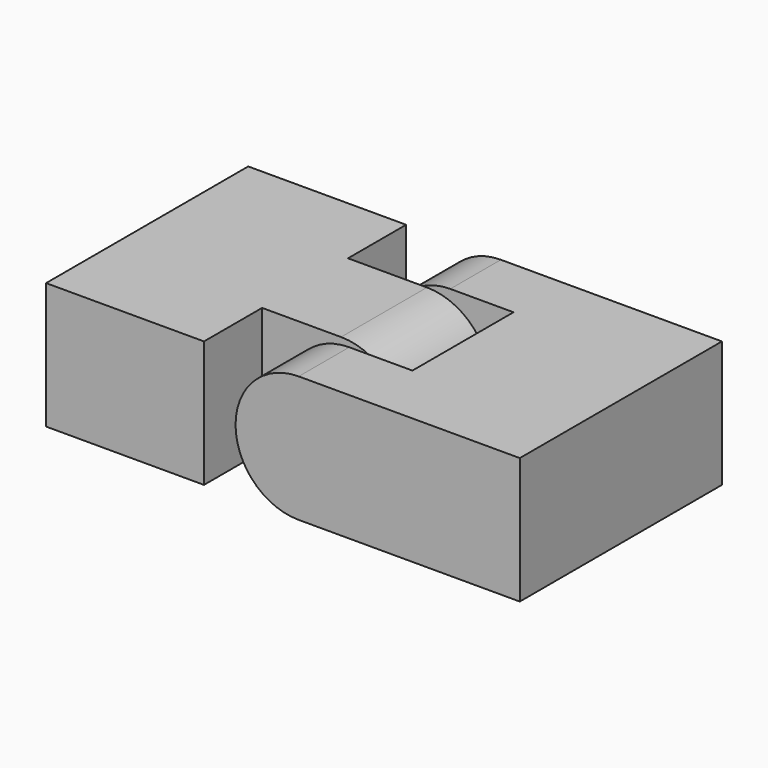
from build123d import *

# Parameters (mm, degrees)
F1_DEPTH = 8
F2_R     = 1.25
F3_DEPTH = 8
F5_DEPTH = 8
F6_R     = 1.8
F7_DEPTH = 6.8
F8_R     = 3.99999
F8_2_R   = 3.99999


# Not quite as in the source:
# - a fillet or chamfer is up to 0.001 mm smaller than in the source, because OpenCascade refuses the exact size


with BuildPart() as f1:
    # F0 (on Top) → F1 (new body)
    with BuildSketch(Plane.XY):
        Polygon((0, 8), (0, 4), (8, 4), (8, -4), (0, -4), (0, -8), (18, -8), (18, 8), align=None)
    extrude(amount=F1_DEPTH)

    # F2 (on face) → F3 (join, through all)
    with BuildSketch(Plane.XZ.offset(-4)):
        with Locations((4, 4)):
            Circle(F2_R)
    extrude(amount=F3_DEPTH)

    # F8 (radius 4 in the source; OpenCascade refuses exactly that, so slightly less here)
    f8_edges = [f1.edges().sort_by_distance(p)[0] for p in [
        (0, 6, 8),
        (0, -6, 8),
        (0, -6, 0),
        (0, 6, 0),
    ]]
    fillet(f8_edges, radius=F8_R)


with BuildPart() as f5:
    # F4 (on face) → F5 (new body, through all)
    with BuildSketch(Plane.XY.offset(8)):
        Polygon((7, -3.4), (7, 3.4), (-2, 3.4), (-2, 8), (-12, 8), (-12, -8), (-2, -8), (-2, -3.4), align=None)
    extrude(amount=-F5_DEPTH)

    # F6 (on face) → F7 (cut, through all)
    with BuildSketch(Plane(origin=(0, 3.4, 0), x_dir=(-1, 0, 0), z_dir=(0, 1, 0))):
        with Locations((-4, 4)):
            Circle(F6_R)
    extrude(amount=-F7_DEPTH, mode=Mode.SUBTRACT)

    # F8#2 (radius 4 in the source; OpenCascade refuses exactly that, so slightly less here)
    f8_2_edges = [f5.edges().sort_by_distance(p)[0] for p in [
        (7, 0, 8),
        (7, 0, 0),
    ]]
    fillet(f8_2_edges, radius=F8_2_R)


solid = Compound([f1.part, f5.part])
